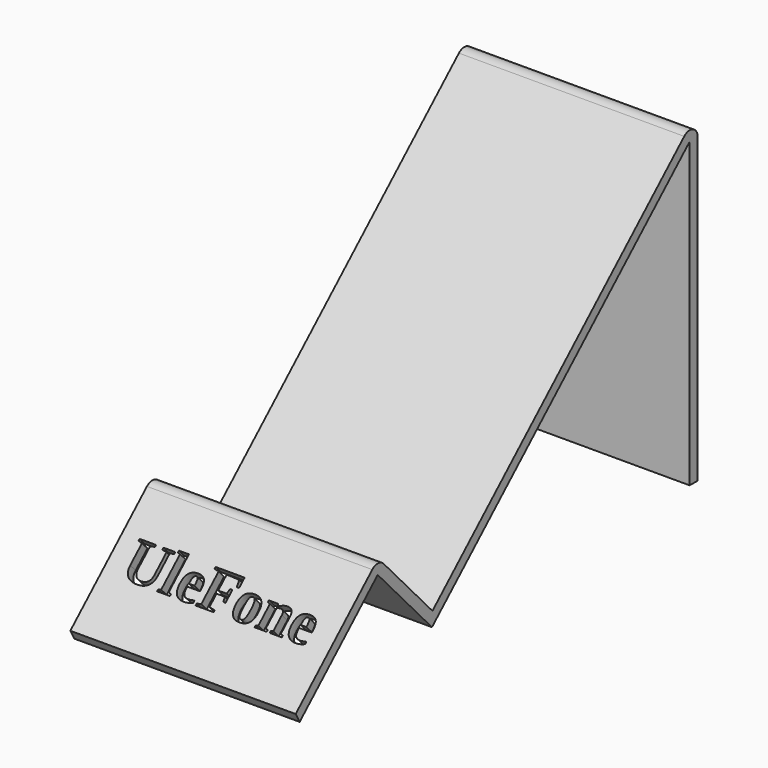
from build123d import *

# Parameters (mm, degrees)
F1_DEPTH     = 45
F2_R         = 2
F3_TEXT_SIZE = 10.5812739297
F4_DEPTH     = 25


# Not quite as in the source:
# - Text() gives the source's letters only with a copy of the font that has no kerning and outlines rounded to 1/6400 em; it was checked with that copy


with BuildPart() as f1:
    # F0 (on Right) → F1 (new body)
    with BuildSketch(Plane.YZ):
        Polygon((66.2096739109, 60.961291658), (0, 0), (-13.5469537018, 14.7132608691), (-34.1455189185, -4.2524743134), (-33.1455189185, -6.0503793824), (-13.6635844185, 11.887239412), (-0.1166307167, -2.8260214571), (64.2096739109, 56.4011939338), (64.2096739109, -4.038708342), (66.2096739109, -4.038708342), align=None)
    extrude(amount=F1_DEPTH)

    # F2
    f2_edges = [f1.edges().sort_by_distance(p)[0] for p in [
        (22.5, 66.209674, 60.961292),
        (22.5, -13.546954, 14.713261),
    ]]
    fillet(f2_edges, radius=F2_R)

    # F3 (on face) → F4 (cut)
    with BuildSketch(Plane(origin=(0, -13.5469537018, 14.7132608691), x_dir=(1, 0, 0), z_dir=(0, -0.6773476851, 0.7356630435))):
        with Locations((3.1542086386, -17.2370344588)):
            Text('UleFone', F3_TEXT_SIZE, font='Tinos', font_style=FontStyle.BOLD, text_align=(TextAlign.LEFT, TextAlign.BOTTOM))
    extrude(amount=-F4_DEPTH, mode=Mode.SUBTRACT)


solid = f1.part
